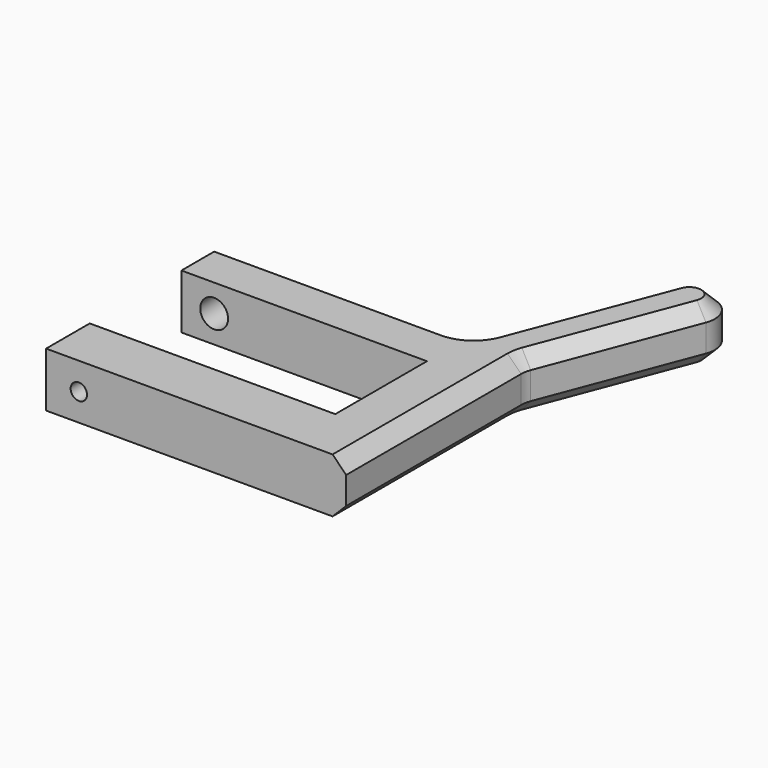
from build123d import *

# Parameters (mm, degrees)
F1_DEPTH       = 10
F3_D           = 5.1
F3_DEPTH       = 20
F3_CSINK_D     = 9.8
F3_CSINK_ANGLE = 90
F3_TIP         = 1.5321945785
F5_D           = 3
F6_T1_DEPTH    = 29.0789805985
F6_T3_DEPTH    = 30.1186834219
F6_T5_DEPTH    = 47.9847156333
F6_T7_DEPTH    = 46.5081880684
F6_T10_ANGLE   = 180
F6_T12_ANGLE   = 180
F6_T14_ANGLE   = 69.1257858818
F6_T16_ANGLE   = 20.8742141182
F6_T18_ANGLE   = 69.1257858818
F6_T20_ANGLE   = 20.8742141182


# Not quite as in the source:
# - a fillet or chamfer that OpenCascade refuses, or shapes differently, is made with other operations: its cross-section is extruded or revolved along the edge and cut away or added


with BuildPart() as f1:
    # F0 (on Top) → F1 (new body)
    with BuildSketch(Plane.XY):
        with BuildLine():
            Line((41.5555081634, 20.5), (0, 20.5))
            Line((0, 20.5), (0, 10.5))
            Line((0, 10.5), (45, 10.5))
            Line((45, 10.5), (45, -10.5))
            Line((45, -10.5), (0, -10.5))
            Line((0, -10.5), (0, -20.5))
            Line((0, -20.5), (45, -20.5))
            Line((45, -20.5), (55, -20.5))
            Line((55, -20.5), (55, 19.5789805985))
            ThreePointArc((55, 19.5789805985), (55.0827282347, 20.4847611382), (55.3281753544, 21.3605682278))
            Line((55.3281753544, 21.3605682278), (65.6895257755, 48.5309478737))
            ThreePointArc((65.6895257755, 48.5309478737), (62.9889896705, 54.5607899764), (56.9591475677, 51.8602538715))
            Line((56.9591475677, 51.8602538715), (46.227332809, 23.7184123708))
            ThreePointArc((46.227332809, 23.7184123708), (44.3920608118, 21.382480228), (41.5555081634, 20.5))
        make_face()
    extrude(amount=F1_DEPTH)

    # F3
    with Locations(Plane(origin=(0, 20.5, 0), x_dir=(-1, 0, 0), z_dir=(0, 1, 0))):
        with Locations((-6, 5)):
            CounterSinkHole(F3_D / 2, F3_CSINK_D / 2, depth=F3_DEPTH, counter_sink_angle=F3_CSINK_ANGLE)
            with Locations((0, 0, -(F3_DEPTH + F3_TIP / 2))):  # 118° drill point
                Cone(0, F3_D / 2, F3_TIP, mode=Mode.SUBTRACT)

    # F5 (through all)
    with Locations(Plane(origin=(0, -10.5, 0), x_dir=(-1, 0, 0), z_dir=(0, 1, 0))):
        with Locations((-6, 5)):
            Hole(F5_D / 2)

    # F6: chamfer of 2.5 on 4 edges, made by hand

    # F6_s2 → F6_t1 (cut)
    with BuildSketch(Plane(origin=(14.1361725075, 37.0690265418, 0), x_dir=(0, 0, 1), z_dir=(0.3563175258, 0.9343649291, 0))):
        Polygon((10, 41.5855618218), (7.5, 44.0855618218), (10, 44.0855618218), align=None)
        Polygon((0, 41.5855618218), (2.5, 44.0855618218), (0, 44.0855618218), align=None)
    extrude(amount=F6_T1_DEPTH, mode=Mode.SUBTRACT)

    # F6_s4 → F6_t3 (cut)
    with BuildSketch(Plane(origin=(24.4975229285, 64.2394061877, 0), x_dir=(0, 0, 1), z_dir=(-0.3563175258, -0.9343649291, 0))):
        Polygon((7.5, -34.7419125306), (10, -37.2419125306), (10, -34.7419125306), align=None)
        Polygon((2.5, -34.7419125306), (0, -37.2419125306), (0, -34.7419125306), align=None)
    extrude(amount=F6_T3_DEPTH, mode=Mode.SUBTRACT)

    # F6_s6 → F6_t5 (cut)
    with BuildSketch(Plane.YZ.offset(-6.4292074699)):
        Polygon((20.5, 7.5), (18, 10), (20.5, 10), align=None)
        Polygon((20.5, 2.5), (18, 0), (20.5, 0), align=None)
    extrude(amount=F6_T5_DEPTH, mode=Mode.SUBTRACT)

    # F6_s8 → F6_t7 (cut)
    with BuildSketch(Plane.XZ.offset(-19.5789805985)):
        Polygon((52.5, 10), (55, 7.5), (55, 10), align=None)
        Polygon((52.5, 0), (55, 2.5), (55, 0), align=None)
    extrude(amount=F6_T7_DEPTH, mode=Mode.SUBTRACT)

    # F6_s9 → F6_t10 (revolve, cut)
    with BuildSketch(Plane(origin=(24.4975229285, 64.2394061877, 0), x_dir=(0, 0, 1), z_dir=(-0.3563175258, -0.9343649291, 0))):
        Polygon((0, -41.5855618218), (2.5, -44.0855618218), (0, -44.0855618218), align=None)
    revolve(axis=Axis((61.3243366716, 50.1956008726, 0), (0, 0, 1)), revolution_arc=F6_T10_ANGLE, mode=Mode.SUBTRACT)

    # F6_s11 → F6_t12 (revolve, cut)
    with BuildSketch(Plane(origin=(24.4975229285, 64.2394061877, 0), x_dir=(0, 0, 1), z_dir=(-0.3563175258, -0.9343649291, 0))):
        Polygon((10, -41.5855618218), (7.5, -44.0855618218), (10, -44.0855618218), align=None)
    revolve(axis=Axis((61.3243366716, 50.1956008726, 10), (0, 0, 1)), revolution_arc=F6_T12_ANGLE, mode=Mode.SUBTRACT)

    # F6_s13 → F6_t14 (revolve, cut)
    with BuildSketch(Plane(origin=(13.7657081698, 36.0975646869, 0), x_dir=(0, 0, 1), z_dir=(0.3563175258, 0.9343649291, 0))):
        Polygon((7.5, 34.7419125306), (10, 37.2419125306), (10, 34.7419125306), align=None)
    revolve(axis=Axis((41.5555081634, 25.5, 10), (0, 0, -1)), revolution_arc=F6_T14_ANGLE, mode=Mode.SUBTRACT)

    # F6_s15 → F6_t16 (revolve, cut)
    with BuildSketch(Plane.XZ.offset(-19.5789805985)):
        Polygon((52.5, 10), (55, 7.5), (55, 10), align=None)
    revolve(axis=Axis((60, 19.5789805985, 10), (0, 0, -1)), revolution_arc=F6_T16_ANGLE, mode=Mode.SUBTRACT)

    # F6_s17 → F6_t18 (revolve, cut)
    with BuildSketch(Plane(origin=(13.7657081698, 36.0975646869, 0), x_dir=(0, 0, 1), z_dir=(0.3563175258, 0.9343649291, 0))):
        Polygon((2.5, 34.7419125306), (0, 37.2419125306), (0, 34.7419125306), align=None)
    revolve(axis=Axis((41.5555081634, 25.5, 0), (0, 0, -1)), revolution_arc=F6_T18_ANGLE, mode=Mode.SUBTRACT)

    # F6_s19 → F6_t20 (revolve, cut)
    with BuildSketch(Plane.XZ.offset(-19.5789805985)):
        Polygon((52.5, 0), (55, 2.5), (55, 0), align=None)
    revolve(axis=Axis((60, 19.5789805985, 0), (0, 0, -1)), revolution_arc=F6_T20_ANGLE, mode=Mode.SUBTRACT)


solid = f1.part
